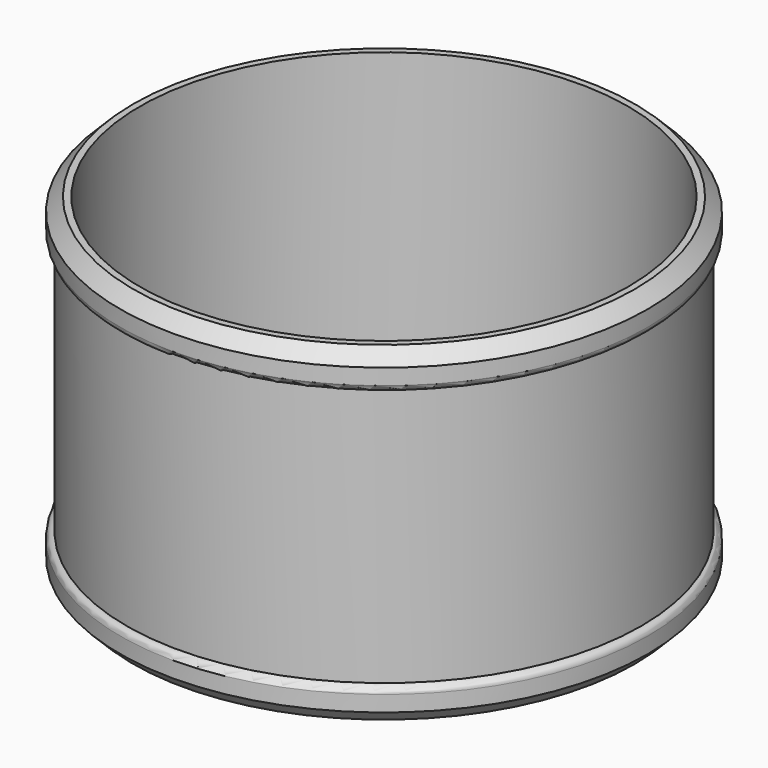
from build123d import *

# Parameters (mm, degrees)
F0_R     = 49.53
F0_R_2   = 46.99
F1_DEPTH = 63.5
F2_R     = 50.8
F2_R_2   = 49.53
F3_DEPTH = 6.858
F4_SIZE  = 2.54
F5_R     = 1.26999
F6_R     = 50.8
F6_R_2   = 49.53
F7_DEPTH = 6.858
F8_SIZE  = 2.54
F9_R     = 1.26999


# Not quite as in the source:
# - a fillet or chamfer is up to 0.001 mm smaller than in the source, because OpenCascade refuses the exact size


with BuildPart() as f1:
    # F0 (on Top) → F1 (new body)
    with BuildSketch(Plane.XY):
        Circle(F0_R)
        Circle(F0_R_2, mode=Mode.SUBTRACT)
    extrude(amount=F1_DEPTH)

    # F2 (on face) → F3 (join)
    with BuildSketch(Plane.XY.offset(63.5)):
        Circle(F2_R)
        Circle(F2_R_2, mode=Mode.SUBTRACT)
    extrude(amount=-F3_DEPTH)

    # F4
    f4_edges = [f1.edges().sort_by_distance(p)[0] for p in [
        (-50.8, 0, 63.5),
    ]]
    chamfer(f4_edges, length=F4_SIZE)

    # F5 (radius 1.27 in the source; OpenCascade refuses exactly that, so slightly less here)
    f5_edges = [f1.edges().sort_by_distance(p)[0] for p in [
        (-50.8, 0, 56.642),
    ]]
    fillet(f5_edges, radius=F5_R)

    # F6 (on face) → F7 (join)
    with BuildSketch(Plane(origin=(0, 0, 0), x_dir=(1, 0, 0), z_dir=(0, 0, -1))):
        Circle(F6_R)
        Circle(F6_R_2, mode=Mode.SUBTRACT)
    extrude(amount=-F7_DEPTH)

    # F8
    f8_edges = [f1.edges().sort_by_distance(p)[0] for p in [
        (-50.8, 0, 0),
    ]]
    chamfer(f8_edges, length=F8_SIZE)

    # F9 (radius 1.27 in the source; OpenCascade refuses exactly that, so slightly less here)
    f9_edges = [f1.edges().sort_by_distance(p)[0] for p in [
        (-50.8, 0, 6.858),
    ]]
    fillet(f9_edges, radius=F9_R)


solid = f1.part
